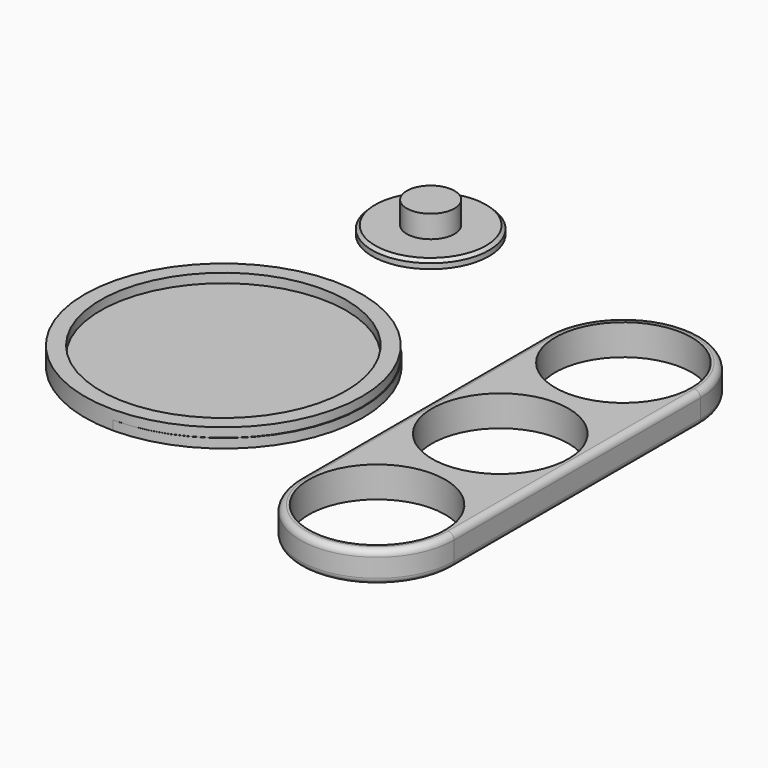
from build123d import *

# Parameters (mm, degrees)
F1_DEPTH  = 5
F2_R      = 11.075
F3_DEPTH  = 25
F4_R      = 22.5
F4_R_2    = 19.945
F5_DEPTH  = 3
F6_R      = 22.5
F7_DEPTH  = 1.5
F8_R      = 9.495
F9_DEPTH  = 1.35
F10_SIZE  = 0.5
F11_R     = 3.875
F12_DEPTH = 3.65
F13_R     = 1


# Not quite as in the source:
# - a feature names something its author has since deleted; it is built from what else it names


with BuildPart() as f1:
    # F0 (on Top) → F1 (new body)
    with BuildSketch(Plane.XY):
        with BuildLine():
            ThreePointArc((0, -12.5), (8.8388347648, -8.8388347648), (12.5, 0))
            ThreePointArc((12.5, 0), (8.8388347677, 8.838834762), (8.1e-09, 12.5))
            ThreePointArc((8.1e-09, 12.5), (-8.838834762, 8.8388347677), (-12.5, 0))
            ThreePointArc((-12.5, 0), (-8.8388347648, -8.8388347648), (0, -12.5))
        make_face()
        with BuildLine():
            Line((12.5, -25), (12.5, 0))
            ThreePointArc((12.5, 0), (8.8388347648, -8.8388347648), (0, -12.5))
            ThreePointArc((0, -12.5), (8.8388347648, -16.1611652352), (12.5, -25))
        make_face()
        with BuildLine():
            ThreePointArc((8.1e-09, 12.5), (8.8388347677, 8.838834762), (12.5, 0))
            Line((12.5, 0), (12.5, 25))
            ThreePointArc((12.5, 25), (8.8388347677, 16.161165238), (8.1e-09, 12.5))
        make_face()
        with BuildLine():
            ThreePointArc((-12.5, 0), (-8.838834762, 8.8388347677), (8.1e-09, 12.5))
            ThreePointArc((8.1e-09, 12.5), (-8.838834762, 16.1611652323), (-12.5, 25))
            Line((-12.5, 25), (-12.5, 0))
        make_face()
        with BuildLine():
            ThreePointArc((-12.5, 25), (-8.838834762, 16.1611652323), (8.1e-09, 12.5))
            ThreePointArc((8.1e-09, 12.5), (8.8388347677, 16.161165238), (12.5, 25))
            ThreePointArc((12.5, 25), (0, 37.5), (-12.5, 25))
        make_face()
        with BuildLine():
            ThreePointArc((-12.5, -25), (-8.8388347648, -16.1611652352), (0, -12.5))
            ThreePointArc((0, -12.5), (-8.8388347648, -8.8388347648), (-12.5, 0))
            Line((-12.5, 0), (-12.5, -25))
        make_face()
        with BuildLine():
            ThreePointArc((12.5, -25), (8.8388347648, -16.1611652352), (0, -12.5))
            ThreePointArc((0, -12.5), (-8.8388347648, -16.1611652352), (-12.5, -25))
            ThreePointArc((-12.5, -25), (0, -37.5), (12.5, -25))
        make_face()
    extrude(amount=F1_DEPTH)

    # F2 (on face) → F3 (cut)
    with BuildSketch(Plane.XY.offset(5)):
        with Locations((0, 25)):
            Circle(F2_R)
        Circle(F2_R)
        with Locations((0, -25)):
            Circle(F2_R)
    extrude(amount=-F3_DEPTH, mode=Mode.SUBTRACT)

    # F13
    f13_edges = [f1.edges().sort_by_distance(p)[0] for p in [
        (-12.5, 0, 5),
        (0, 37.5, 5),
        (0, -37.5, 5),
        (0, -37.5, 0),
        (12.5, 0, 0),
        (0, 37.5, 0),
        (-12.5, 0, 0),
    ]]
    fillet(f13_edges, radius=F13_R)


with BuildPart() as f5:
    # F4 (on Top) → F5 (new body)
    with BuildSketch(Plane.XY):
        with Locations((-44.9528545141, 0)):
            Circle(F4_R)
        with Locations((-44.9528545141, 0)):
            Circle(F4_R_2, mode=Mode.SUBTRACT)
    extrude(amount=F5_DEPTH)

    # F6 (on face) → F7 (join)
    with BuildSketch(Plane.XY):
        with Locations((-44.8220527387, 0)):
            Circle(F6_R)
    extrude(amount=F7_DEPTH)


with BuildPart() as f9:
    # F8 (on Top) → F9 (new body)
    with BuildSketch(Plane.XY):
        with Locations((-47.0260679722, 44.662322849)):
            Circle(F8_R)
    extrude(amount=F9_DEPTH)

    # F10
    f10_edges = [f9.edges().sort_by_distance(p)[0] for p in [
        (-56.521068, 44.662323, 1.35),
    ]]
    chamfer(f10_edges, length=F10_SIZE)

    # F11 (on face) → F12 (join)
    with BuildSketch(Plane.XY.offset(1.35)):
        with Locations((-47.0260679722, 44.662322849)):
            Circle(F11_R)
    extrude(amount=F12_DEPTH)


solid = Compound([f1.part, f5.part, f9.part])
